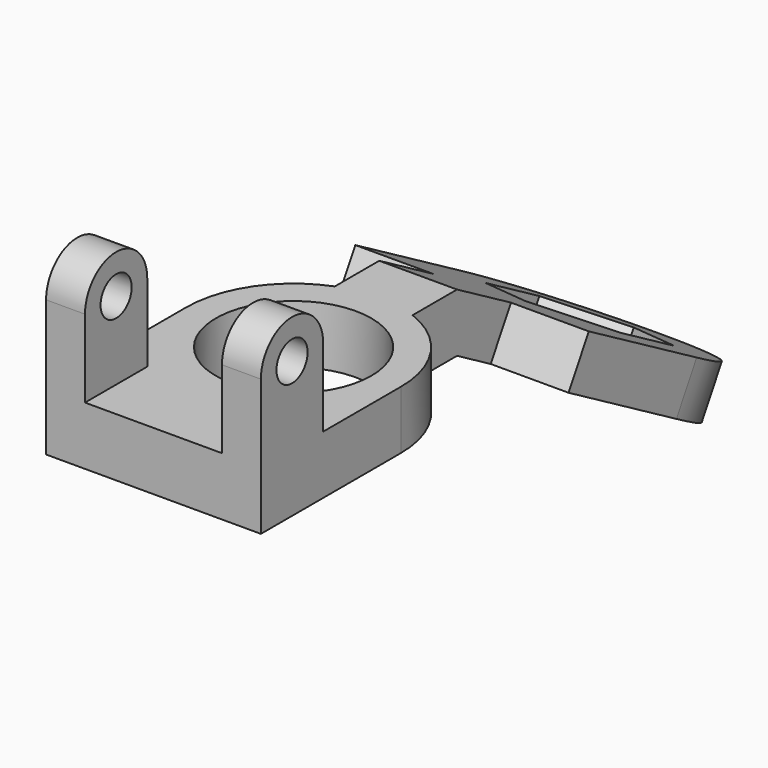
from build123d import *

# Parameters (mm, degrees)
F0_R          = 25.4
F1_DEPTH      = 19.05
F2_R          = 6.35
F3_DEPTH      = 12.7
F5_DEPTH      = 25.4
F5_DEPTH_BACK = 50.8
F6_W          = 25.4
F6_H          = 25.4
F7_DEPTH      = 25.4
F9_DEPTH      = 115.8426897829


# Not quite as in the source:
# - a pattern or mirror of a feature is missing from the dataset's text; its kind, count and spacing are read off the source's solid


with BuildPart() as f1:
    # F0 (on Top) → F1 (new body)
    with BuildSketch(Plane.XY):
        with BuildLine():
            Line((-35.052, -28.575), (35.052, -28.575))
            Line((35.052, -28.575), (35.052, 28.575))
            ThreePointArc((35.052, 28.575), (28.9292508026, 48.3674518946), (12.7, 61.2453643077))
            Line((12.7, 61.2453643077), (12.7, 79.375))
            Line((12.7, 79.375), (-12.7, 79.375))
            Line((-12.7, 79.375), (-12.7, 61.2453643077))
            ThreePointArc((-12.7, 61.2453643077), (-28.9292508026, 48.3674518946), (-35.052, 28.575))
            Line((-35.052, 28.575), (-35.052, -28.575))
        make_face()
        with Locations((0, 28.575)):
            Circle(F0_R, mode=Mode.SUBTRACT)
    extrude(amount=F1_DEPTH)

    # F2 (on face) → F3 (join)
    with BuildSketch(Plane(origin=(-35.052, 0, 0), x_dir=(0, -1, 0), z_dir=(-1, 0, 0))):
        with BuildLine():
            Line((3.175, 19.05), (28.575, 19.05))
            Line((28.575, 19.05), (28.575, 44.45))
            ThreePointArc((28.575, 44.45), (15.875, 57.15), (3.175, 44.45))
            Line((3.175, 44.45), (3.175, 19.05))
        make_face()
        with Locations((15.875, 44.45)):
            Circle(F2_R, mode=Mode.SUBTRACT)
    f3 = extrude(amount=-F3_DEPTH)

    # F3_copies: F3 across plane
    add(f3.mirror(Plane(origin=(0, 0, 0), x_dir=(0, 0, 1), z_dir=(1, 0, 0))))

    # F4 (on face) → F5 (join, two sides)
    with BuildSketch(Plane(origin=(-12.7, 0, 0), x_dir=(0, -1, 0), z_dir=(-1, 0, 0))) as f5_sk:
        Polygon((-79.375, 0), (-79.375, 19.05), (-178.3617036526, -38.1), (-170.1128116815, -52.3875), align=None)
    extrude(amount=F5_DEPTH)
    extrude(f5_sk.sketch, amount=-F5_DEPTH_BACK)

    # F6 (on face) → F7 (cut)
    with BuildSketch(Plane(origin=(0, 28.092641971, 48.6578832127), x_dir=(1, 0, 0), z_dir=(0, 0.5, 0.8660254038))):
        with Locations((25.4, 71.9157664254)):
            Rectangle(F6_W, F6_H)
        with Locations((-25.4, 71.9157664254)):
            Rectangle(F6_W, F6_H)
        with BuildLine():
            ThreePointArc((-38.1, 135.4157664254), (-26.9407683632, 162.3565347886), (0, 173.5157664254))
            Line((0, 173.5157664254), (-38.1, 173.5157664254))
            Line((-38.1, 173.5157664254), (-38.1, 135.4157664254))
        make_face()
        with BuildLine():
            ThreePointArc((0, 173.5157664254), (26.9407683632, 162.3565347886), (38.1, 135.4157664254))
            Line((38.1, 135.4157664254), (38.1, 173.5157664254))
            Line((38.1, 173.5157664254), (0, 173.5157664254))
        make_face()
    extrude(amount=-F7_DEPTH, mode=Mode.SUBTRACT)

    # F8 (on face) → F9 (cut, through all)
    with BuildSketch(Plane(origin=(0, 28.092641971, 48.6578832127), x_dir=(1, 0, 0), z_dir=(0, 0.5, 0.8660254038))):
        Polygon((21.9970411706, 148.1157664254), (-4.0856e-06, 160.8157664254), (-21.9970493417, 148.1157664254), (-21.9970493417, 122.7157664254), (-4.0856e-06, 110.0157664254), (21.9970411706, 122.7157664254), align=None)
    extrude(amount=-F9_DEPTH, mode=Mode.SUBTRACT)


solid = f1.part
